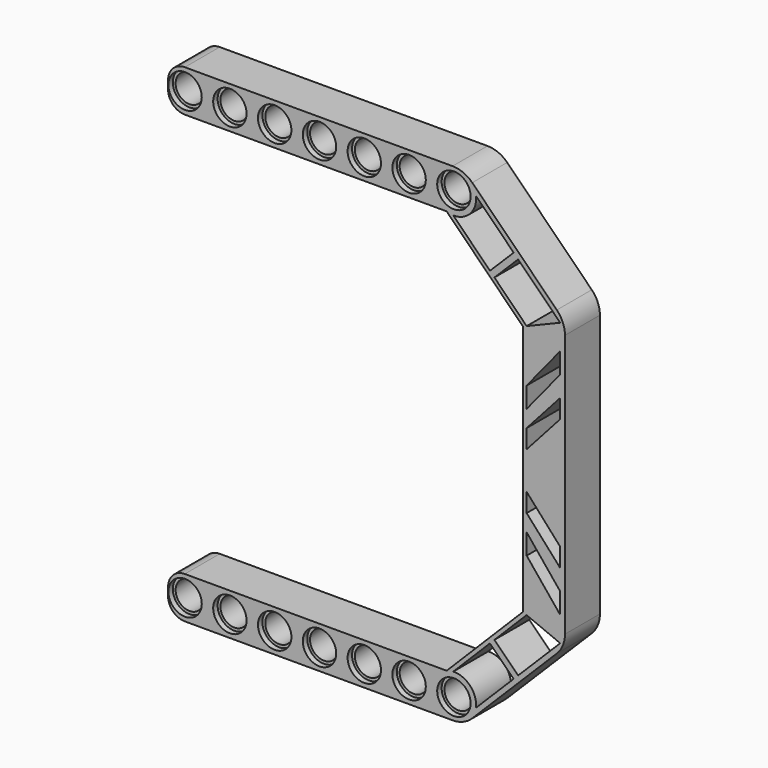
from build123d import *

# Parameters (mm, degrees)
F0_R     = 3
F0_R_2   = 2.499
F1_DEPTH = 3.925
F2_R     = 3
F3_R     = 5
F4_R     = 3
F5_DEPTH = 1
F6_R     = 3
F6_R_2   = 2.499
F7_DEPTH = 1


# Not quite as in the source:
# - ends of sketch curves that miss each other by under 0.0002 mm in the source are joined


with BuildPart() as f1:
    # F0 (on Front) → F1 (new body, symmetric)
    with BuildSketch(Plane.XZ):
        Polygon((18.9613047033, 18.3160076926), (17.5273123959, 19.75), (-35.65, 19.75), (-35.65, 12.25), (14.4, 12.25), (28.1, -1.5000000006), (28.15, -19.7499999994), (28.15, -28.3999999994), (28.1, -46.65), (14.4, -60.4), (-35.65, -60.4), (-35.65, -67.9), (17.5273123959, -67.9), (18.9613047033, -66.4660076926), (35.65, -49.7773123959), (35.65, -28.4), (35.65, -19.75), (35.65, 1.6273123959), align=None)
        with Locations((-32.6, -64.15)):
            Circle(F0_R, mode=Mode.SUBTRACT)
        with Locations((-24.55, -64.15)):
            Circle(F0_R, mode=Mode.SUBTRACT)
        with Locations((-16.5, -64.15)):
            Circle(F0_R, mode=Mode.SUBTRACT)
        with Locations((-8.45, -64.15)):
            Circle(F0_R, mode=Mode.SUBTRACT)
        with Locations((-0.4, -64.15)):
            Circle(F0_R, mode=Mode.SUBTRACT)
        with Locations((7.65, -64.15)):
            Circle(F0_R, mode=Mode.SUBTRACT)
        with Locations((15.7, -64.15)):
            Circle(F0_R, mode=Mode.SUBTRACT)
        with BuildLine():
            ThreePointArc((19.6811007558, -64.5383771008), (18.6244738475, -61.4209978536), (15.5875186741, -60.1515818189))
            Line((15.5875186741, -60.1515818189), (22.1713217449, -53.5437502697))
            Line((22.1713217449, -53.5437502697), (22.9770950322, -52.735036204))
            Line((22.9770950322, -52.735036204), (28.7653917701, -46.9256142955))
            Line((28.7653917701, -46.9256142955), (34.7959320067, -49.4235458499))
            Line((34.7959320067, -49.4235458499), (27.2385163812, -56.9809614754))
            Line((27.2385163812, -56.9809614754), (26.4235246659, -57.7959531907))
            Line((26.4235246659, -57.7959531907), (19.6811007558, -64.5383771008))
        make_face(mode=Mode.SUBTRACT)
        Polygon((34.7959320067, -41.2253109008), (34.7959320067, -44.9256142955), (28.7681314859, -37.525), (28.7681314859, -33.8246890992), align=None, mode=Mode.SUBTRACT)
        Polygon((34.7959320067, -37.525), (28.7681314859, -30.7990158793), (28.7681314859, -27.436514941), (34.7959320067, -34.1624990617), align=None, mode=Mode.SUBTRACT)
        with Locations((-32.6, 16)):
            Circle(F0_R, mode=Mode.SUBTRACT)
        with Locations((-24.55, 16)):
            Circle(F0_R, mode=Mode.SUBTRACT)
        with Locations((-16.5, 16)):
            Circle(F0_R, mode=Mode.SUBTRACT)
        with Locations((-8.45, 16)):
            Circle(F0_R, mode=Mode.SUBTRACT)
        with Locations((-0.4, 16)):
            Circle(F0_R, mode=Mode.SUBTRACT)
        Polygon((28.7681314859, -20.7134831825), (28.7690151327, -17.3499982396), (34.7959320067, -10.625), (34.7959320067, -13.9874990617), (28.7685732445, -20.7129902561), align=None, mode=Mode.SUBTRACT)
        Polygon((28.7681314859, -10.625), (28.7698990648, -10.6228298581), (34.7959320067, -3.2243781985), (34.7959320067, -6.9246890992), (28.7694127753, -14.3237377999), (28.7698987796, -10.625), align=None, mode=Mode.SUBTRACT)
        with Locations((7.65, 16)):
            Circle(F0_R, mode=Mode.SUBTRACT)
        with Locations((15.7, 16)):
            Circle(F0_R, mode=Mode.SUBTRACT)
        with BuildLine():
            Line((22.176455222, 5.388598057), (15.5875186741, 12.0015818188))
            ThreePointArc((15.5875186741, 12.0015818188), (18.6244738475, 13.2709978536), (19.6811007558, 16.3883771008))
            Line((19.6811007558, 16.3883771008), (26.4364128886, 9.6330649683))
            Line((26.4364128886, 9.6330649683), (27.2385163814, 8.8309614755))
            Line((27.2385163814, 8.8309614755), (34.795932007, 1.2735458502))
            Line((34.795932007, 1.2735458502), (28.7653917699, -1.2243857048))
            Line((28.7653917699, -1.2243857048), (22.977095032, 4.5850362039))
            Line((22.977095032, 4.5850362039), (22.176455222, 5.388598057))
        make_face(mode=Mode.SUBTRACT)
        with Locations((-32.6, 16)):
            Circle(F0_R)
        with Locations((-32.6, 16)):
            Circle(F0_R_2, mode=Mode.SUBTRACT)
        with Locations((-24.55, 16)):
            Circle(F0_R)
        with Locations((-24.55, 16)):
            Circle(F0_R_2, mode=Mode.SUBTRACT)
        with Locations((-16.5, 16)):
            Circle(F0_R)
        with Locations((-16.5, 16)):
            Circle(F0_R_2, mode=Mode.SUBTRACT)
        with Locations((-0.4, 16)):
            Circle(F0_R)
        with Locations((-0.4, 16)):
            Circle(F0_R_2, mode=Mode.SUBTRACT)
        with Locations((7.65, 16)):
            Circle(F0_R)
        with Locations((7.65, 16)):
            Circle(F0_R_2, mode=Mode.SUBTRACT)
        with Locations((-8.45, 16)):
            Circle(F0_R)
        with Locations((-8.45, 16)):
            Circle(F0_R_2, mode=Mode.SUBTRACT)
        with Locations((15.7, 16)):
            Circle(F0_R)
        with Locations((15.7, 16)):
            Circle(F0_R_2, mode=Mode.SUBTRACT)
        with Locations((7.65, -64.15)):
            Circle(F0_R)
        with Locations((7.65, -64.15)):
            Circle(F0_R_2, mode=Mode.SUBTRACT)
        with Locations((15.7, -64.15)):
            Circle(F0_R)
        with Locations((15.7, -64.15)):
            Circle(F0_R_2, mode=Mode.SUBTRACT)
        with Locations((-0.4, -64.15)):
            Circle(F0_R)
        with Locations((-0.4, -64.15)):
            Circle(F0_R_2, mode=Mode.SUBTRACT)
        with Locations((-8.45, -64.15)):
            Circle(F0_R)
        with Locations((-8.45, -64.15)):
            Circle(F0_R_2, mode=Mode.SUBTRACT)
        with Locations((-16.5, -64.15)):
            Circle(F0_R)
        with Locations((-16.5, -64.15)):
            Circle(F0_R_2, mode=Mode.SUBTRACT)
        with Locations((-24.55, -64.15)):
            Circle(F0_R)
        with Locations((-24.55, -64.15)):
            Circle(F0_R_2, mode=Mode.SUBTRACT)
        with Locations((-32.6, -64.15)):
            Circle(F0_R)
        with Locations((-32.6, -64.15)):
            Circle(F0_R_2, mode=Mode.SUBTRACT)
        Polygon((22.9770950322, -52.735036204), (22.1713217449, -53.5437502697), (26.4235246659, -57.7959531907), (27.2385163812, -56.9809614754), align=None)
        Polygon((26.4364128886, 9.6330649683), (22.176455222, 5.388598057), (22.977095032, 4.5850362039), (27.2385163814, 8.8309614755), align=None)
    extrude(amount=F1_DEPTH, both=True)

    # F2
    f2_edges = [f1.edges().sort_by_distance(p)[0] for p in [
        (-35.65, 0, 19.75),
        (-35.65, 0, 12.25),
        (-35.65, 0, -60.4),
        (-35.65, 0, -67.9),
    ]]
    fillet(f2_edges, radius=F2_R)

    # F3
    f3_edges = [f1.edges().sort_by_distance(p)[0] for p in [
        (35.65, 0, 1.627312),
        (17.527312, 0, 19.75),
        (35.65, 0, -49.777312),
        (17.527312, 0, -67.9),
    ]]
    fillet(f3_edges, radius=F3_R)

    # F4 (on face) → F5 (cut)
    with BuildSketch(Plane.XZ.offset(3.925)):
        with Locations((-24.55, 16)):
            Circle(F4_R)
        with Locations((-16.5, 16)):
            Circle(F4_R)
        with Locations((-8.45, 16)):
            Circle(F4_R)
        with Locations((-0.4, 16)):
            Circle(F4_R)
        with Locations((7.65, 16)):
            Circle(F4_R)
        with Locations((15.7, 16)):
            Circle(F4_R)
        with Locations((-32.6, 16)):
            Circle(F4_R)
        with Locations((-32.6, -64.15)):
            Circle(F4_R)
        with Locations((-24.55, -64.15)):
            Circle(F4_R)
        with Locations((-16.5, -64.15)):
            Circle(F4_R)
        with Locations((-8.45, -64.15)):
            Circle(F4_R)
        with Locations((-0.4, -64.15)):
            Circle(F4_R)
        with Locations((7.65, -64.15)):
            Circle(F4_R)
        with Locations((15.7, -64.15)):
            Circle(F4_R)
    extrude(amount=-F5_DEPTH, mode=Mode.SUBTRACT)

    # F6 (on face) → F7 (cut)
    with BuildSketch(Plane(origin=(0, 3.925, 0), x_dir=(-1, 0, 0), z_dir=(0, 1, 0))):
        with Locations((-15.7, 16)):
            Circle(F6_R)
        with Locations((-15.7, 16)):
            Circle(F6_R_2, mode=Mode.SUBTRACT)
        with Locations((-7.65, 16)):
            Circle(F6_R)
        with Locations((-7.65, 16)):
            Circle(F6_R_2, mode=Mode.SUBTRACT)
        with Locations((0.4, 16)):
            Circle(F6_R)
        with Locations((0.4, 16)):
            Circle(F6_R_2, mode=Mode.SUBTRACT)
        with Locations((8.45, 16)):
            Circle(F6_R)
        with Locations((8.45, 16)):
            Circle(F6_R_2, mode=Mode.SUBTRACT)
        with Locations((16.5, 16)):
            Circle(F6_R)
        with Locations((16.5, 16)):
            Circle(F6_R_2, mode=Mode.SUBTRACT)
        with Locations((24.55, 16)):
            Circle(F6_R)
        with Locations((24.55, 16)):
            Circle(F6_R_2, mode=Mode.SUBTRACT)
        with Locations((32.6, 16)):
            Circle(F6_R)
        with Locations((32.6, 16)):
            Circle(F6_R_2, mode=Mode.SUBTRACT)
        with Locations((-15.7, -64.15)):
            Circle(F6_R)
        with Locations((-15.7, -64.15)):
            Circle(F6_R_2, mode=Mode.SUBTRACT)
        with Locations((-7.65, -64.15)):
            Circle(F6_R)
        with Locations((-7.65, -64.15)):
            Circle(F6_R_2, mode=Mode.SUBTRACT)
        with Locations((0.4, -64.15)):
            Circle(F6_R)
        with Locations((0.4, -64.15)):
            Circle(F6_R_2, mode=Mode.SUBTRACT)
        with Locations((8.45, -64.15)):
            Circle(F6_R)
        with Locations((8.45, -64.15)):
            Circle(F6_R_2, mode=Mode.SUBTRACT)
        with Locations((16.5, -64.15)):
            Circle(F6_R)
        with Locations((16.5, -64.15)):
            Circle(F6_R_2, mode=Mode.SUBTRACT)
        with Locations((24.55, -64.15)):
            Circle(F6_R)
        with Locations((24.55, -64.15)):
            Circle(F6_R_2, mode=Mode.SUBTRACT)
        with Locations((32.6, -64.15)):
            Circle(F6_R)
        with Locations((32.6, -64.15)):
            Circle(F6_R_2, mode=Mode.SUBTRACT)
    extrude(amount=-F7_DEPTH, mode=Mode.SUBTRACT)


solid = f1.part
